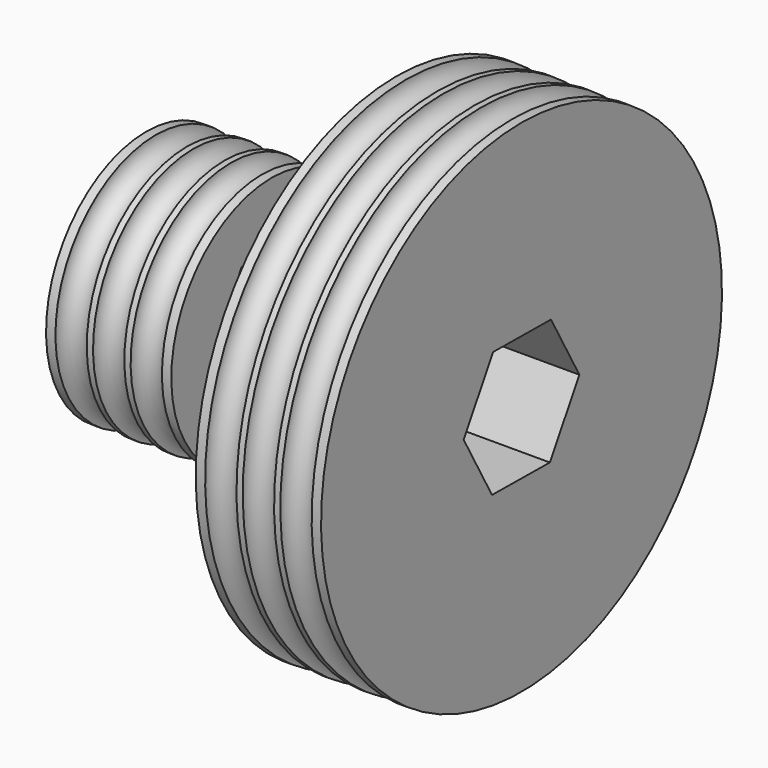
from build123d import *

# Parameters (mm, degrees)
F3_DEPTH = 13.3328129599
F7_DEPTH = 25.4


with BuildPart() as f1:
    # F0 (on Front) → F1 (revolve)
    with BuildSketch(Plane.XZ):
        with BuildLine():
            ThreePointArc((4.7593129599, 24.6499903677), (3.1718129599, 23.0624903677), (1.5843129599, 24.6499903677))
            Line((1.5843129599, 24.6499903677), (0.6318129599, 24.6499903677))
            Line((0.6318129599, 24.6499903677), (0.6318129599, 11.9499903677))
            Line((0.6318129599, 11.9499903677), (13.3318129599, 11.9499903677))
            Line((13.3318129599, 11.9499903677), (13.3318129599, 24.6499903677))
            Line((13.3318129599, 24.6499903677), (12.3793129599, 24.6499903677))
            ThreePointArc((12.3793129599, 24.6499903677), (10.7918129599, 23.0624903677), (9.2043129599, 24.6499903677))
            Line((9.2043129599, 24.6499903677), (8.5693129599, 24.6499903677))
            ThreePointArc((8.5693129599, 24.6499903677), (6.9818129599, 23.0624903677), (5.3943129599, 24.6499903677))
            Line((5.3943129599, 24.6499903677), (4.7593129599, 24.6499903677))
        make_face()
    revolve(axis=Axis((6.9818129599, 0, 11.9499903677), (-1, 0, 0)))

    # F2 (on Right) → F3 (cut, through all)
    with BuildSketch(Plane.YZ):
        Polygon((3.8137593804, 5.6875169967), (7.33034072, 12.1215661895), (3.5165813396, 18.3840395605), (-3.8137593804, 18.2124637387), (-7.33034072, 11.7784145458), (-3.5165813396, 5.5159411749), align=None)
    extrude(amount=F3_DEPTH, mode=Mode.SUBTRACT)


with BuildPart() as f5:
    # F4 (on Front) → F5 (revolve)
    with BuildSketch(Plane.XZ):
        with BuildLine():
            ThreePointArc((30.0949377739, 37.814297089), (28.5074377739, 36.226797089), (26.9199377739, 37.814297089))
            Line((26.9199377739, 37.814297089), (25.9674377739, 37.814297089))
            Line((25.9674377739, 37.814297089), (25.9674377739, 12.414297089))
            Line((25.9674377739, 12.414297089), (38.6674377739, 12.414297089))
            Line((38.6674377739, 12.414297089), (38.6674377739, 37.814297089))
            Line((38.6674377739, 37.814297089), (37.7149377739, 37.814297089))
            ThreePointArc((37.7149377739, 37.814297089), (36.1274377739, 36.226797089), (34.5399377739, 37.814297089))
            Line((34.5399377739, 37.814297089), (33.9049377739, 37.814297089))
            ThreePointArc((33.9049377739, 37.814297089), (32.3174377739, 36.226797089), (30.7299377739, 37.814297089))
            Line((30.7299377739, 37.814297089), (30.0949377739, 37.814297089))
        make_face()
    revolve(axis=Axis((32.3174377739, 0, 12.414297089), (1, 0, 0)))

    # F6 (on face) → F7 (cut)
    with BuildSketch(Plane.YZ.offset(38.6674377739)):
        Polygon((7.3318888043, 12.3322002234), (3.7370423733, 18.7228506184), (-3.5948464309, 18.804947484), (-7.3318888043, 12.4963939546), (-3.7370423733, 6.1057435596), (3.5948464309, 6.023646694), align=None)
    extrude(amount=-F7_DEPTH, mode=Mode.SUBTRACT)


solid = Compound([f1.part, f5.part])
